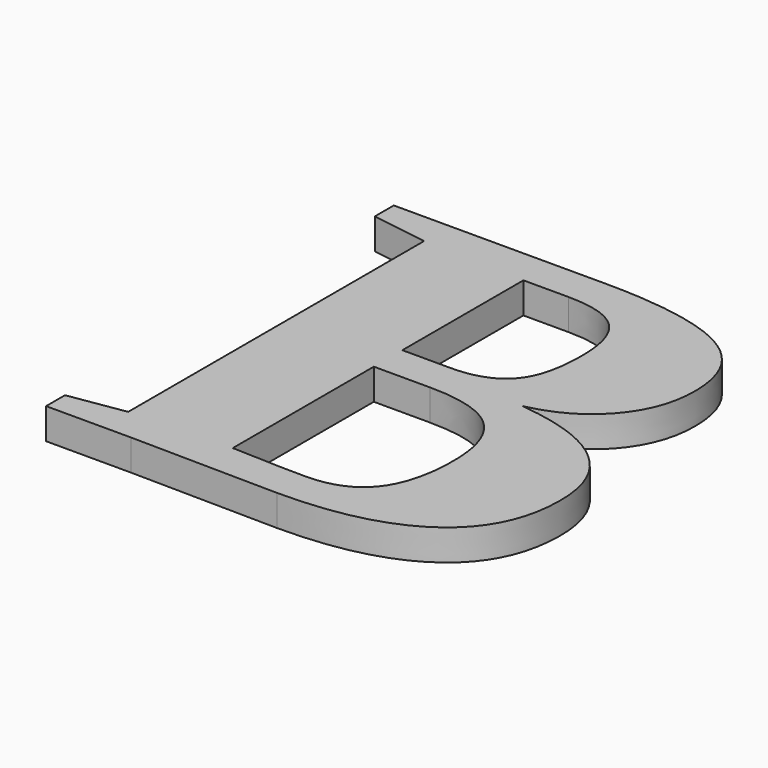
from build123d import *

# Parameters (mm, degrees)
F0_TEXT_SIZE = 109.0122438553
F1_DEPTH     = 5.08


# Not quite as in the source:
# - Text() gives the source's letters only with a copy of the font that has no kerning and outlines rounded to 1/6400 em; it was checked with that copy


with BuildPart() as f1:
    # F0 (on Top) → F1 (new body)
    with BuildSketch(Plane.XY):
        with Locations((-35.5547592044, -38.7412831187)):
            Text('B', F0_TEXT_SIZE, font='Tinos', font_style=FontStyle.BOLD, text_align=(TextAlign.LEFT, TextAlign.BOTTOM))
    extrude(amount=F1_DEPTH)


solid = f1.part
